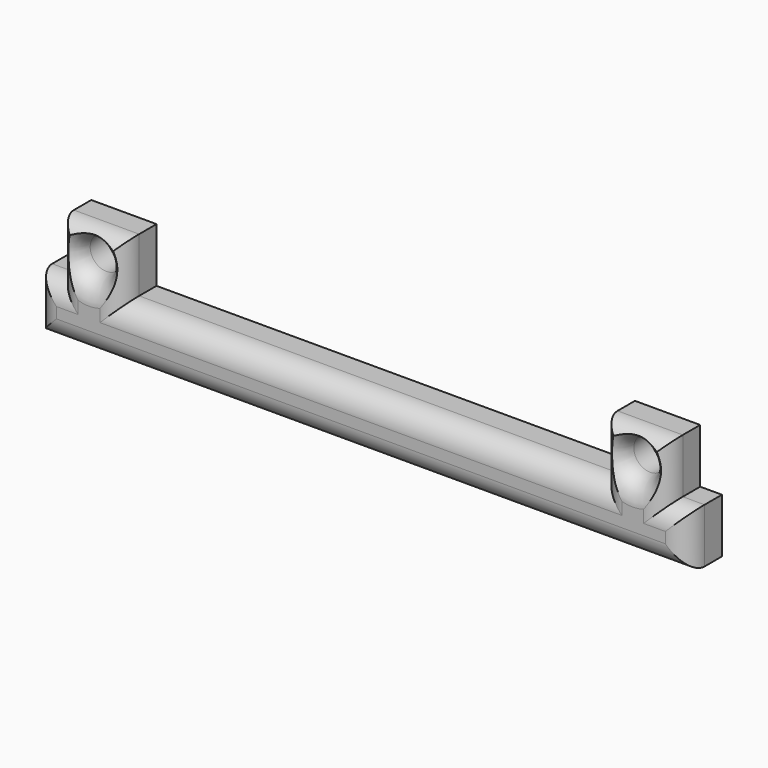
from build123d import *

# Parameters (mm, degrees)
F0_R         = 1.5
F1_DEPTH     = 4
F2_T1_DEPTH  = 15
F2_T3_DEPTH  = 70
F2_T5_DEPTH  = 7
F2_T7_DEPTH  = 10
F2_T9_DEPTH  = 16
F2_T11_DEPTH = 44
F2_T13_DEPTH = 16
F2_T15_DEPTH = 7
F2_T25_DEPTH = 12
F2_T29_DEPTH = 15
F2_T36_DEPTH = 15
F2_T40_DEPTH = 49
F2_T47_DEPTH = 49
F2_T51_DEPTH = 15
F2_T58_DEPTH = 15
F2_T62_DEPTH = 12


# Not quite as in the source:
# - a fillet or chamfer that OpenCascade refuses, or shapes differently, is made with other operations: its cross-section is extruded or revolved along the edge and cut away or added


with BuildPart() as f1:
    # F0 (on Front) → F1 (new body)
    with BuildSketch(Plane.XZ):
        Polygon((-55, 5), (-55, 0), (5, 0), (5, 5), (3, 5), (3, 10), (-3, 10), (-3, 5), (-47, 5), (-47, 10), (-53, 10), (-53, 5), align=None)
        with Locations((-50, 7.5)):
            Circle(F0_R, mode=Mode.SUBTRACT)
        with Locations((0, 7.5)):
            Circle(F0_R, mode=Mode.SUBTRACT)
    extrude(amount=F1_DEPTH)

    # F2: fillet of radius 2 on 14 edges, made by hand

    # F2_s2 → F2_t1 (cut)
    with BuildSketch(Plane.XY.offset(-5)):
        with BuildLine():
            ThreePointArc((-55, -2), (-54.4142135624, -3.4142135624), (-53, -4))
            Line((-53, -4), (-55, -4))
            Line((-55, -4), (-55, -2))
        make_face()
        with BuildLine():
            ThreePointArc((5, -2), (4.4142135624, -3.4142135624), (3, -4))
            Line((3, -4), (5, -4))
            Line((5, -4), (5, -2))
        make_face()
    extrude(amount=F2_T1_DEPTH, mode=Mode.SUBTRACT)

    # F2_s4 → F2_t3 (cut)
    with BuildSketch(Plane.YZ.offset(-60)):
        with BuildLine():
            ThreePointArc((-2, 0), (-3.4142135624, 0.5857864376), (-4, 2))
            Line((-4, 2), (-4, 0))
            Line((-4, 0), (-2, 0))
        make_face()
    extrude(amount=F2_T3_DEPTH, mode=Mode.SUBTRACT)

    # F2_s6 → F2_t5 (cut)
    with BuildSketch(Plane.YZ.offset(3)):
        with BuildLine():
            ThreePointArc((-2, 5), (-3.4142135624, 4.4142135624), (-4, 3))
            Line((-4, 3), (-4, 5))
            Line((-4, 5), (-2, 5))
        make_face()
    extrude(amount=F2_T5_DEPTH, mode=Mode.SUBTRACT)

    # F2_s8 → F2_t7 (cut)
    with BuildSketch(Plane.XY.offset(5)):
        with BuildLine():
            ThreePointArc((3, -2), (2.4142135624, -3.4142135624), (1, -4))
            Line((1, -4), (3, -4))
            Line((3, -4), (3, -2))
        make_face()
        with BuildLine():
            ThreePointArc((-3, -2), (-2.4142135624, -3.4142135624), (-1, -4))
            Line((-1, -4), (-3, -4))
            Line((-3, -4), (-3, -2))
        make_face()
        with BuildLine():
            ThreePointArc((-47, -2), (-47.5857864376, -3.4142135624), (-49, -4))
            Line((-49, -4), (-47, -4))
            Line((-47, -4), (-47, -2))
        make_face()
        with BuildLine():
            ThreePointArc((-53, -2), (-52.4142135624, -3.4142135624), (-51, -4))
            Line((-51, -4), (-53, -4))
            Line((-53, -4), (-53, -2))
        make_face()
    extrude(amount=F2_T7_DEPTH, mode=Mode.SUBTRACT)

    # F2_s10 → F2_t9 (cut)
    with BuildSketch(Plane.YZ.offset(-8)):
        with BuildLine():
            ThreePointArc((-2, 10), (-3.4142135624, 9.4142135624), (-4, 8))
            Line((-4, 8), (-4, 10))
            Line((-4, 10), (-2, 10))
        make_face()
    extrude(amount=F2_T9_DEPTH, mode=Mode.SUBTRACT)

    # F2_s12 → F2_t11 (cut)
    with BuildSketch(Plane.YZ.offset(-47)):
        with BuildLine():
            ThreePointArc((-2, 5), (-3.4142135624, 4.4142135624), (-4, 3))
            Line((-4, 3), (-4, 5))
            Line((-4, 5), (-2, 5))
        make_face()
    extrude(amount=F2_T11_DEPTH, mode=Mode.SUBTRACT)

    # F2_s14 → F2_t13 (cut)
    with BuildSketch(Plane.YZ.offset(-58)):
        with BuildLine():
            ThreePointArc((-2, 10), (-3.4142135624, 9.4142135624), (-4, 8))
            Line((-4, 8), (-4, 10))
            Line((-4, 10), (-2, 10))
        make_face()
    extrude(amount=F2_T13_DEPTH, mode=Mode.SUBTRACT)

    # F2_s16 → F2_t15 (cut)
    with BuildSketch(Plane.YZ.offset(-60)):
        with BuildLine():
            ThreePointArc((-2, 5), (-3.4142135624, 4.4142135624), (-4, 3))
            Line((-4, 3), (-4, 5))
            Line((-4, 5), (-2, 5))
        make_face()
    extrude(amount=F2_T15_DEPTH, mode=Mode.SUBTRACT)

    # F2_s17 → F2_t18 (revolve, cut)
    with BuildSketch(Plane.XY.offset(7.5)):
        with BuildLine():
            ThreePointArc((-48.5, -2), (-47.9142135624, -3.4142135624), (-46.5, -4))
            Line((-46.5, -4), (-48.5, -4))
            Line((-48.5, -4), (-48.5, -2))
        make_face()
    revolve(axis=Axis((-50, -4, 7.5), (0, -1, 0)), mode=Mode.SUBTRACT)

    # F2_s19 → F2_t20 (revolve, cut)
    with BuildSketch(Plane.XY.offset(7.5)):
        with BuildLine():
            ThreePointArc((1.5, -2), (2.0857864376, -3.4142135624), (3.5, -4))
            Line((3.5, -4), (1.5, -4))
            Line((1.5, -4), (1.5, -2))
        make_face()
    revolve(axis=Axis((0, -4, 7.5), (0, -1, 0)), mode=Mode.SUBTRACT)


with BuildPart() as f2_tool23:
    # F2_s24 → F2_t25 (new body)
    with BuildSketch(Plane.YZ.offset(10)):
        with BuildLine():
            ThreePointArc((-2, 5), (-3.4142135624, 4.4142135624), (-4, 3))
            Line((-4, 3), (-4, 5))
            Line((-4, 5), (-2, 5))
        make_face()
    extrude(amount=-F2_T25_DEPTH)

    split(bisect_by=Plane.YZ.offset(3), keep=Keep.BOTTOM)


with BuildPart() as f2_tool27:
    # F2_s28 → F2_t29 (new body)
    with BuildSketch(Plane.XY):
        with BuildLine():
            ThreePointArc((3, -2), (2.4142135624, -3.4142135624), (1, -4))
            Line((1, -4), (3, -4))
            Line((3, -4), (3, -2))
        make_face()
    extrude(amount=F2_T29_DEPTH)

    split(bisect_by=Plane.XY.offset(5), keep=Keep.BOTTOM)


with BuildPart() as f2_tool23_1:
    add(f2_tool23.part)

    # F2_t31: intersect F2_tool27
    add(f2_tool27.part, mode=Mode.INTERSECT)


with BuildPart() as f1_1:
    add(f1.part)

    # F2_t21: cut F2_tool23
    add(f2_tool23_1.part, mode=Mode.SUBTRACT)


with BuildPart() as f2_tool34:
    # F2_s35 → F2_t36 (new body)
    with BuildSketch(Plane.XY.offset(15)):
        with BuildLine():
            ThreePointArc((-3, -2), (-2.4142135624, -3.4142135624), (-1, -4))
            Line((-1, -4), (-3, -4))
            Line((-3, -4), (-3, -2))
        make_face()
    extrude(amount=-F2_T36_DEPTH)

    split(bisect_by=Plane.XY.offset(5), keep=Keep.BOTTOM)


with BuildPart() as f2_tool38:
    # F2_s39 → F2_t40 (new body)
    with BuildSketch(Plane.YZ.offset(2)):
        with BuildLine():
            ThreePointArc((-2, 5), (-3.4142135624, 4.4142135624), (-4, 3))
            Line((-4, 3), (-4, 5))
            Line((-4, 5), (-2, 5))
        make_face()
    extrude(amount=-F2_T40_DEPTH)

    split(bisect_by=Plane.YZ.offset(-3), keep=Keep.TOP)


with BuildPart() as f2_tool34_1:
    add(f2_tool34.part)

    # F2_t42: intersect F2_tool38
    add(f2_tool38.part, mode=Mode.INTERSECT)


with BuildPart() as f1_2:
    add(f1_1.part)

    # F2_t32: cut F2_tool34
    add(f2_tool34_1.part, mode=Mode.SUBTRACT)


with BuildPart() as f2_tool45:
    # F2_s46 → F2_t47 (new body)
    with BuildSketch(Plane.YZ.offset(-3)):
        with BuildLine():
            ThreePointArc((-2, 5), (-3.4142135624, 4.4142135624), (-4, 3))
            Line((-4, 3), (-4, 5))
            Line((-4, 5), (-2, 5))
        make_face()
    extrude(amount=-F2_T47_DEPTH)

    split(bisect_by=Plane.YZ.offset(-47), keep=Keep.BOTTOM)


with BuildPart() as f2_tool49:
    # F2_s50 → F2_t51 (new body)
    with BuildSketch(Plane.XY):
        with BuildLine():
            ThreePointArc((-47, -2), (-47.5857864376, -3.4142135624), (-49, -4))
            Line((-49, -4), (-47, -4))
            Line((-47, -4), (-47, -2))
        make_face()
    extrude(amount=F2_T51_DEPTH)

    split(bisect_by=Plane.XY.offset(5), keep=Keep.BOTTOM)


with BuildPart() as f2_tool45_1:
    add(f2_tool45.part)

    # F2_t53: intersect F2_tool49
    add(f2_tool49.part, mode=Mode.INTERSECT)


with BuildPart() as f1_3:
    add(f1_2.part)

    # F2_t43: cut F2_tool45
    add(f2_tool45_1.part, mode=Mode.SUBTRACT)


with BuildPart() as f2_tool56:
    # F2_s57 → F2_t58 (new body)
    with BuildSketch(Plane.XY.offset(15)):
        with BuildLine():
            ThreePointArc((-53, -2), (-52.4142135624, -3.4142135624), (-51, -4))
            Line((-51, -4), (-53, -4))
            Line((-53, -4), (-53, -2))
        make_face()
    extrude(amount=-F2_T58_DEPTH)

    split(bisect_by=Plane.XY.offset(5), keep=Keep.BOTTOM)


with BuildPart() as f2_tool60:
    # F2_s61 → F2_t62 (new body)
    with BuildSketch(Plane.YZ.offset(-48)):
        with BuildLine():
            ThreePointArc((-2, 5), (-3.4142135624, 4.4142135624), (-4, 3))
            Line((-4, 3), (-4, 5))
            Line((-4, 5), (-2, 5))
        make_face()
    extrude(amount=-F2_T62_DEPTH)

    split(bisect_by=Plane.YZ.offset(-53), keep=Keep.TOP)


with BuildPart() as f2_tool56_1:
    add(f2_tool56.part)

    # F2_t64: intersect F2_tool60
    add(f2_tool60.part, mode=Mode.INTERSECT)


with BuildPart() as f1_4:
    add(f1_3.part)

    # F2_t54: cut F2_tool56
    add(f2_tool56_1.part, mode=Mode.SUBTRACT)


solid = f1_4.part
